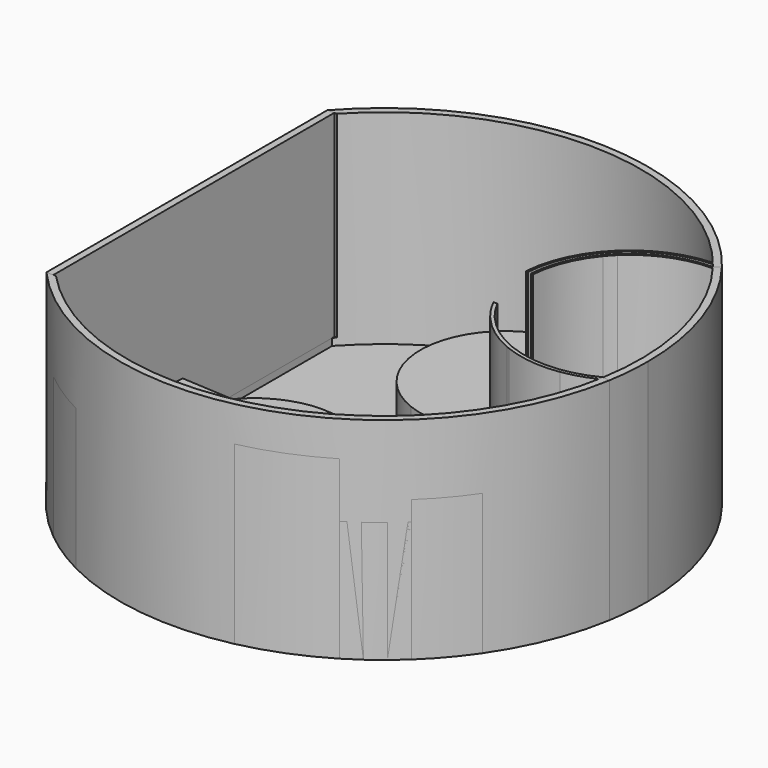
from build123d import *

# Parameters (mm, degrees)
F0_R         = 37.5
F1_DEPTH     = 30
F3_DEPTH     = 28
F8_T         = 1
F8_T3_DEPTH  = 51.8898787331
F9_DEPTH     = 20
F10_DEPTH    = 20
F11_DEPTH    = 25
F12_DEPTH    = 25
F13_DEPTH    = 30
F14_DEPTH    = 30
F15_DEPTH    = 20
F16_DEPTH    = 20
F17_W        = 49.8898787331
F17_H        = 28
F18_DEPTH    = 1.3551748111
F19_DEPTH    = 1
F22_DEPTH    = 5
F23_DEPTH    = 10
F24_DEPTH    = 9
F25_DEPTH    = 8
F26_DEPTH    = 30
F27_DEPTH    = 6
F28_DEPTH    = 4
F21_R        = 1
F29_DEPTH    = 10.5
F30_DEPTH    = 11
F31_DEPTH    = 10
F32_DEPTH    = 8
F33_DEPTH    = 25
F34_DEPTH    = 25
F35_T2_ANGLE = 246.718091376


# Not quite as in the source:
# - a fillet or chamfer that OpenCascade refuses, or shapes differently, is made with other operations: its cross-section is extruded or revolved along the edge and cut away or added
# - a shell that OpenCascade refuses in one call is made with other operations: the cavity is built on its own and cut out


with BuildPart() as f1:
    # F0 (on Top) → F1 (new body)
    with BuildSketch(Plane.XY):
        Circle(F0_R)
    extrude(amount=-F1_DEPTH)

    # F2 (on face) → F3 (cut)
    with BuildSketch(Plane.XY):
        with BuildLine():
            Line((-28, -24.9449393665), (-28, 24.9449393665))
            ThreePointArc((-28, 24.9449393665), (-37.5, 0), (-28, -24.9449393665))
        make_face()
    extrude(amount=-F3_DEPTH, mode=Mode.SUBTRACT)

    # F8: shell of thickness 1, made by hand


with BuildPart() as f8_core1:
    # F8_t2: copy of F1
    add(f1.part)

    # the walls: a layer under each face that stays
    f8_faces = [f8_core1.faces().sort_by_distance(p)[0] for p in [
        (18.75, 32.4759526419, -25),
        (-28, 0, -14),
        (-32.75, 0, -28),
        (0, 0, -30),
    ]]
    thicken(f8_faces, amount=-F8_T, mode=Mode.SUBTRACT)

    # F8_s4 → F8_t3 (cut)
    with BuildSketch(Plane.XZ.offset(-25.9449393665)):
        Polygon((-28.01, -27.99), (-27, -28), (-27, -29), (-28, -29), align=None)
    extrude(amount=F8_T3_DEPTH, mode=Mode.SUBTRACT)


with BuildPart() as f1_1:
    add(f1.part)

    # what is left inside the walls is the cavity
    f8_cavity = [f8_core1.part.solids().sort_by_distance(p)[0] for p in [
        (36.49, 0, -19.333333),
    ]]
    add(f8_cavity, mode=Mode.SUBTRACT)

    # F6 (on face) → F9 (cut)
    with BuildSketch(Plane(origin=(0, 0, -30), x_dir=(1, 0, 0), z_dir=(0, 0, -1))):
        with BuildLine():
            ThreePointArc((-16.953998922, 33.4486460197), (-20.4251291644, 31.4493894793), (-23.6632020109, 29.0912851313))
            Line((-23.6632020109, 29.0912851313), (-23.0321832906, 28.3155175278))
            ThreePointArc((-23.0321832906, 28.3155175278), (-19.8804590533, 30.6107390931), (-16.501892284, 32.5566821259))
            Line((-16.501892284, 32.5566821259), (-16.953998922, 33.4486460197))
        make_face()
    extrude(amount=-F9_DEPTH, mode=Mode.SUBTRACT)

    # F7 (on face) → F11 (cut)
    with BuildSketch(Plane(origin=(0, 0, -30), x_dir=(1, 0, 0), z_dir=(0, 0, -1))):
        with BuildLine():
            ThreePointArc((19.3711654827, 32.1093124785), (13.8934103709, 34.8313529491), (8.046001078, 36.6266551387))
            Line((8.046001078, 36.6266551387), (6.8659209199, 31.2547457184))
            ThreePointArc((6.8659209199, 31.2547457184), (11.2981173091, 29.9391473704), (15.494474725, 27.9985937682))
            Line((15.494474725, 27.9985937682), (19.3711654827, 32.1093124785))
        make_face()
    extrude(amount=-F11_DEPTH, mode=Mode.SUBTRACT)

    # F7 (on face) → F13 (cut)
    with BuildSketch(Plane(origin=(0, 0, -30), x_dir=(1, 0, 0), z_dir=(0, 0, -1))):
        with BuildLine():
            Line((28.9052016216, -22.2876494771), (29.6971249537, -22.8982700107))
            ThreePointArc((29.6971249537, -22.8982700107), (35.49571936, -12.0956152021), (37.5, 0))
            ThreePointArc((37.5, 0), (37.3706102437, 3.1124732958), (36.9833338658, 6.2034680763))
            Line((36.9833338658, 6.2034680763), (35.9971116293, 6.038042261))
            ThreePointArc((35.9971116293, 6.038042261), (35.4071146726, -8.8648875097), (28.9052016216, -22.2876494771))
        make_face()
    extrude(amount=-F13_DEPTH, mode=Mode.SUBTRACT)

    # F7 (on face) → F15 (cut)
    with BuildSketch(Plane(origin=(0, 0, -30), x_dir=(1, 0, 0), z_dir=(0, 0, -1))):
        with BuildLine():
            ThreePointArc((30.9299683404, 21.2034680763), (28.4918045576, 24.3816954507), (25.7285399775, 27.2817197153))
            Line((25.7285399775, 27.2817197153), (25.0424455781, 26.5542071896))
            ThreePointArc((25.0424455781, 26.5542071896), (27.7320231027, 23.7315169054), (30.1051691846, 20.638042261))
            Line((30.1051691846, 20.638042261), (30.9299683404, 21.2034680763))
        make_face()
    extrude(amount=-F15_DEPTH, mode=Mode.SUBTRACT)

    # F17 (on face) → F18 (cut, through all)
    with BuildSketch(Plane(origin=(-28, 0, 0), x_dir=(0, -1, 0), z_dir=(-1, 0, 0))):
        with Locations((0, -14)):
            Rectangle(F17_W, F17_H)
    extrude(amount=-F18_DEPTH, mode=Mode.SUBTRACT)


with BuildPart() as f10:
    # F6 (on face) → F10 (new body)
    with BuildSketch(Plane(origin=(0, 0, -30), x_dir=(1, 0, 0), z_dir=(0, 0, -1))):
        with BuildLine():
            ThreePointArc((-16.953998922, 33.4486460197), (-20.4251291644, 31.4493894793), (-23.6632020109, 29.0912851313))
            Line((-23.6632020109, 29.0912851313), (-23.0321832906, 28.3155175278))
            ThreePointArc((-23.0321832906, 28.3155175278), (-19.8804590533, 30.6107390931), (-16.501892284, 32.5566821259))
            Line((-16.501892284, 32.5566821259), (-16.953998922, 33.4486460197))
        make_face()
    extrude(amount=-F10_DEPTH)


with BuildPart() as f12:
    # F7 (on face) → F12 (new body)
    with BuildSketch(Plane(origin=(0, 0, -30), x_dir=(1, 0, 0), z_dir=(0, 0, -1))):
        with BuildLine():
            ThreePointArc((19.3711654827, 32.1093124785), (13.8934103709, 34.8313529491), (8.046001078, 36.6266551387))
            Line((8.046001078, 36.6266551387), (6.8659209199, 31.2547457184))
            ThreePointArc((6.8659209199, 31.2547457184), (11.2981173091, 29.9391473704), (15.494474725, 27.9985937682))
            Line((15.494474725, 27.9985937682), (19.3711654827, 32.1093124785))
        make_face()
    extrude(amount=-F12_DEPTH)


with BuildPart() as f14:
    # F7 (on face) → F14 (new body)
    with BuildSketch(Plane(origin=(0, 0, -30), x_dir=(1, 0, 0), z_dir=(0, 0, -1))):
        with BuildLine():
            Line((28.9052016216, -22.2876494771), (29.6971249537, -22.8982700107))
            ThreePointArc((29.6971249537, -22.8982700107), (35.49571936, -12.0956152021), (37.5, 0))
            ThreePointArc((37.5, 0), (37.3706102437, 3.1124732958), (36.9833338658, 6.2034680763))
            Line((36.9833338658, 6.2034680763), (35.9971116293, 6.038042261))
            ThreePointArc((35.9971116293, 6.038042261), (35.4071146726, -8.8648875097), (28.9052016216, -22.2876494771))
        make_face()
    extrude(amount=-F14_DEPTH)


with BuildPart() as f16:
    # F7 (on face) → F16 (new body)
    with BuildSketch(Plane(origin=(0, 0, -30), x_dir=(1, 0, 0), z_dir=(0, 0, -1))):
        with BuildLine():
            ThreePointArc((30.9299683404, 21.2034680763), (28.4918045576, 24.3816954507), (25.7285399775, 27.2817197153))
            Line((25.7285399775, 27.2817197153), (25.0424455781, 26.5542071896))
            ThreePointArc((25.0424455781, 26.5542071896), (27.7320231027, 23.7315169054), (30.1051691846, 20.638042261))
            Line((30.1051691846, 20.638042261), (30.9299683404, 21.2034680763))
        make_face()
    extrude(amount=-F16_DEPTH)


with BuildPart() as f19:
    # F17 (on face) → F19 (new body)
    with BuildSketch(Plane(origin=(-28, 0, 0), x_dir=(0, -1, 0), z_dir=(-1, 0, 0))):
        with Locations((0, -14)):
            Rectangle(F17_W, F17_H)
    extrude(amount=-F19_DEPTH)


with BuildPart() as f22:
    # F20 (on face) → F22 (new body)
    with BuildSketch(Plane(origin=(0, 0, -30), x_dir=(1, 0, 0), z_dir=(0, 0, -1))):
        with BuildLine():
            ThreePointArc((-6.2381378075, -12.6227108912), (-8.6582514015, -33.9201866001), (10.2955201074, -23.9104929502))
            ThreePointArc((10.2955201074, -23.9104929502), (9.929155312, -20.9530515767), (8.8522099626, -18.1744059794))
            ThreePointArc((8.8522099626, -18.1744059794), (2.3602210357, -12.5358422681), (-6.2381378075, -12.6227108912))
        make_face()
    extrude(amount=-F22_DEPTH)


with BuildPart() as f22b:
    # F20 (on face) → F22, piece 2 (new body)
    with BuildSketch(Plane(origin=(0, 0, -30), x_dir=(1, 0, 0), z_dir=(0, 0, -1))):
        with BuildLine():
            ThreePointArc((-2.6626795947, 11.4102402329), (-24.8517523428, 10.5323016938), (-9.1514433618, -5.1720296642))
            ThreePointArc((-9.1514433618, -5.1720296642), (-3.5554076268, -0.7180191141), (-1.4451012766, 6.1157523948))
            ThreePointArc((-1.4451012766, 6.1157523948), (-1.7534174258, 8.8320963728), (-2.6626795947, 11.4102402329))
        make_face()
    extrude(amount=-F22_DEPTH)


with BuildPart() as f22c:
    # F20 (on face) → F22, piece 3 (new body)
    with BuildSketch(Plane(origin=(0, 0, -30), x_dir=(1, 0, 0), z_dir=(0, 0, -1))):
        with BuildLine():
            Line((9.0313370609, 9.5891463299), (9.0313370609, 11.6807336927))
            ThreePointArc((9.0313370609, 11.6807336927), (6.9616271493, 12.092424591), (5.2070118097, 13.2648210787))
            Line((5.2070118097, 13.2648210787), (3.728036202, 11.785845471))
            ThreePointArc((3.728036202, 11.785845471), (6.1612113182, 10.1600498361), (9.0313370609, 9.5891463299))
        make_face()
    extrude(amount=-F22_DEPTH)


with BuildPart() as f22d:
    # F20 (on face) → F22, piece 4 (new body)
    with BuildSketch(Plane(origin=(0, 0, -30), x_dir=(1, 0, 0), z_dir=(0, 0, -1))):
        with BuildLine():
            Line((12.8556623122, 13.2648210787), (14.3346379198, 11.785845471))
            ThreePointArc((14.3346379198, 11.785845471), (15.9604335548, 14.2190205872), (16.5313370609, 17.0891463299))
            Line((16.5313370609, 17.0891463299), (14.4397496982, 17.0891463299))
            ThreePointArc((14.4397496982, 17.0891463299), (14.0280587999, 15.0194364182), (12.8556623122, 13.2648210787))
        make_face()
    extrude(amount=-F22_DEPTH)


with BuildPart() as f22e:
    # F20 (on face) → F22, piece 5 (new body)
    with BuildSketch(Plane(origin=(0, 0, -30), x_dir=(1, 0, 0), z_dir=(0, 0, -1))):
        with BuildLine():
            ThreePointArc((9.0313370609, 22.4975589671), (11.1010469726, 22.0858680688), (12.8556623122, 20.9134715811))
            Line((12.8556623122, 20.9134715811), (14.3346379198, 22.3924471888))
            ThreePointArc((14.3346379198, 22.3924471888), (11.9014628037, 24.0182428237), (9.0313370609, 24.5891463299))
            Line((9.0313370609, 24.5891463299), (9.0313370609, 22.4975589671))
        make_face()
    extrude(amount=-F22_DEPTH)


with BuildPart() as f22f:
    # F20 (on face) → F22, piece 6 (new body)
    with BuildSketch(Plane(origin=(0, 0, -30), x_dir=(1, 0, 0), z_dir=(0, 0, -1))):
        with BuildLine():
            ThreePointArc((3.6229244237, 17.0891463299), (4.034615322, 19.1588562416), (5.2070118097, 20.9134715811))
            Line((5.2070118097, 20.9134715811), (3.728036202, 22.3924471888))
            ThreePointArc((3.728036202, 22.3924471888), (2.1022405671, 19.9592720726), (1.5313370609, 17.0891463299))
            Line((1.5313370609, 17.0891463299), (3.6229244237, 17.0891463299))
        make_face()
    extrude(amount=-F22_DEPTH)


with BuildPart() as f23:
    # F20 (on face) → F23 (new body)
    with BuildSketch(Plane(origin=(0, 0, -30), x_dir=(1, 0, 0), z_dir=(0, 0, -1))):
        with BuildLine():
            ThreePointArc((14.0313370609, 17.0891463299), (7.9107331096, 21.9619531991), (4.5336383473, 14.9049516772))
            ThreePointArc((4.5336383473, 14.9049516772), (10.1519410123, 12.2163394607), (14.0313370609, 17.0891463299))
        make_face()
    extrude(amount=-F23_DEPTH)


with BuildPart() as f24:
    # F21 (on face) → F24 (new body)
    with BuildSketch(Plane(origin=(0, 0, -30), x_dir=(1, 0, 0), z_dir=(0, 0, -1))):
        with BuildLine():
            ThreePointArc((-13.6560176054, 7.6129946), (-12.5370872916, 7.2080835014), (-12.0651012766, 6.1157523948))
            ThreePointArc((-12.0651012766, 6.1157523948), (-12.472770206, 5.0877383715), (-13.4741850526, 4.6185101832))
            Line((-13.4741850526, 4.6185101832), (-1.4694765849, 5.3474664352))
            Line((-1.4694765849, 5.3474664352), (-1.6513092498, 8.3419508452))
            Line((-1.6513092498, 8.3419508452), (-13.6560176054, 7.6129946))
        make_face()
    extrude(amount=-F24_DEPTH)


with BuildPart() as f24b:
    # F21 (on face) → F24, piece 2 (new body)
    with BuildSketch(Plane(origin=(0, 0, -30), x_dir=(1, 0, 0), z_dir=(0, 0, -1))):
        with BuildLine():
            ThreePointArc((-13.4741850526, 4.6185101832), (-15.0623434851, 6.0248361184), (-13.6560176054, 7.6129946))
            Line((-13.6560176054, 7.6129946), (-25.6607259684, 6.8840383544))
            Line((-25.6607259684, 6.8840383544), (-25.4788933035, 3.8895539444))
            Line((-25.4788933035, 3.8895539444), (-13.4741850526, 4.6185101832))
        make_face()
    extrude(amount=-F24_DEPTH)


with BuildPart() as f25:
    # F21 (on face) → F25 (new body)
    with BuildSketch(Plane(origin=(0, 0, -30), x_dir=(1, 0, 0), z_dir=(0, 0, -1))):
        with BuildLine():
            ThreePointArc((-13.4741850526, 4.6185101832), (-12.472770206, 5.0877383715), (-12.0651012766, 6.1157523948))
            ThreePointArc((-12.0651012766, 6.1157523948), (-12.5370872916, 7.2080835014), (-13.6560176054, 7.6129946))
            ThreePointArc((-13.6560176054, 7.6129946), (-15.0623434851, 6.0248361184), (-13.4741850526, 4.6185101832))
        make_face()
    extrude(amount=-F25_DEPTH)


with BuildPart() as f26:
    # F21 (on face) → F26 (new body)
    with BuildSketch(Plane(origin=(0, 0, -30), x_dir=(1, 0, 0), z_dir=(0, 0, -1))):
        with BuildLine():
            Line((17.3724938816, 2.8304197599), (17.0417262015, 2.4334684989))
            ThreePointArc((17.0417262015, 2.4334684989), (16.0363047925, 1.0321677906), (15.1927880508, -0.4721577696))
            Line((15.1927880508, -0.4721577696), (15.7749208381, -0.4269615575))
            ThreePointArc((15.7749208381, -0.4269615575), (16.5120762756, 0.8478783333), (17.3706855082, 2.0442917535))
            ThreePointArc((17.3706855082, 2.0442917535), (17.5291229842, 2.2402246522), (17.6908293548, 2.4334684989))
            ThreePointArc((17.6908293548, 2.4334684989), (20.2548787509, 4.8158309177), (23.3012175242, 6.5391475102))
            ThreePointArc((23.3012175242, 6.5391475102), (23.5343220983, 6.634826098), (23.7690009761, 6.7265755334))
            ThreePointArc((23.7690009761, 6.7265755334), (29.9565305021, 7.6871850383), (35.9971116293, 6.038042261))
            Line((35.9971116293, 6.038042261), (35.8888105379, 6.6515620853))
            ThreePointArc((35.8888105379, 6.6515620853), (33.7046086375, 7.5152810001), (31.4149776339, 8.039054017))
            ThreePointArc((31.4149776339, 8.039054017), (27.3986887439, 8.1157854532), (23.4975592214, 7.157843592))
            Line((23.4975592214, 7.157843592), (23.019151936, 6.9626410533))
            ThreePointArc((23.019151936, 6.9626410533), (19.9595995404, 5.2193283623), (17.3724938816, 2.8304197599))
        make_face()
    extrude(amount=-F26_DEPTH)


with BuildPart() as f26b:
    # F21 (on face) → F26, piece 2 (new body)
    with BuildSketch(Plane(origin=(0, 0, -30), x_dir=(1, 0, 0), z_dir=(0, 0, -1))):
        with BuildLine():
            ThreePointArc((18.9043539971, -17.8658754357), (18.9379553483, -18.1056753585), (18.9756990746, -18.3448582694))
            ThreePointArc((18.9756990746, -18.3448582694), (23.5775248273, -21.2302434033), (28.9052016216, -22.2876494771))
            Line((28.9052016216, -22.2876494771), (29.1132550673, -21.9890924211))
            ThreePointArc((29.1132550673, -21.9890924211), (23.6081987695, -20.9193659017), (18.9043539971, -17.8658754357))
        make_face()
        with BuildLine():
            ThreePointArc((14.1582603233, -8.4501833766), (15.2874731924, -13.1069748149), (17.8275811834, -17.1700622615))
            ThreePointArc((17.8275811834, -17.1700622615), (17.8109483721, -16.9218415031), (17.7984344878, -16.673379035))
            ThreePointArc((17.7984344878, -16.673379035), (15.4889985638, -12.8090231025), (14.4573602182, -8.4269615575))
            Line((14.4573602182, -8.4269615575), (14.1582603233, -8.4501833766))
        make_face()
        with BuildLine():
            ThreePointArc((17.7984344878, -16.673379035), (17.8109483721, -16.9218415031), (17.8275811834, -17.1700622615))
            Line((17.8275811834, -17.1700622615), (18.9756990746, -18.3448582694))
            ThreePointArc((18.9756990746, -18.3448582694), (18.9379553483, -18.1056753585), (18.9043539971, -17.8658754357))
            ThreePointArc((18.9043539971, -17.8658754357), (18.3348896843, -17.2849335397), (17.7984344878, -16.673379035))
        make_face()
    extrude(amount=-F26_DEPTH)


with BuildPart() as f26c:
    # F21 (on face) → F26, piece 3 (new body)
    with BuildSketch(Plane(origin=(0, 0, -30), x_dir=(1, 0, 0), z_dir=(0, 0, -1))):
        with BuildLine():
            Line((28.2867848352, -23.0674620122), (28.5205850004, -22.7777573794))
            ThreePointArc((28.5205850004, -22.7777573794), (18.3702197288, -18.4621489283), (13.6597604985, -8.4888864085))
            Line((13.6597604985, -8.4888864085), (13.3606606036, -8.5121082276))
            ThreePointArc((13.3606606036, -8.5121082276), (18.0823472399, -18.6009920186), (28.2867848352, -23.0674620122))
        make_face()
    extrude(amount=-F26_DEPTH)


with BuildPart() as f27:
    # F21 (on face) → F27 (new body)
    with BuildSketch(Plane(origin=(0, 0, -30), x_dir=(1, 0, 0), z_dir=(0, 0, -1))):
        with BuildLine():
            ThreePointArc((36.4690616321, -1.5025124541), (23.3259292755, -4.4017029134), (17.7984344878, -16.673379035))
            ThreePointArc((17.7984344878, -16.673379035), (18.3348896843, -17.2849335397), (18.9043539971, -17.8658754357))
            ThreePointArc((18.9043539971, -17.8658754357), (23.5577123643, -5.5144047174), (36.4128165524, -2.521267682))
            Line((36.4128165524, -2.521267682), (36.4690616321, -1.5025124541))
        make_face()
    extrude(amount=-F27_DEPTH)


with BuildPart() as f28:
    # F21 (on face) → F28 (new body)
    with BuildSketch(Plane(origin=(0, 0, -30), x_dir=(1, 0, 0), z_dir=(0, 0, -1))):
        with BuildLine():
            Line((33.6939781628, 0.0919253308), (33.384353908, 4.0799239292))
            Line((33.384353908, 4.0799239292), (30.3933549592, 3.8477057381))
            ThreePointArc((30.3933549592, 3.8477057381), (28.5541677874, 1.6988943115), (30.7029792141, -0.1402928603))
            Line((30.7029792141, -0.1402928603), (33.6939781628, 0.0919253308))
        make_face()
    extrude(amount=-F28_DEPTH)


with BuildPart() as f29:
    # F21 (on face) → F29 (new body)
    with BuildSketch(Plane(origin=(0, 0, -30), x_dir=(1, 0, 0), z_dir=(0, 0, -1))):
        with Locations((28.4533989432, 12.6025223553)):
            Circle(F21_R)
    extrude(amount=-F29_DEPTH)


with BuildPart() as f29b:
    # F21 (on face) → F29, piece 2 (new body)
    with BuildSketch(Plane(origin=(0, 0, -30), x_dir=(1, 0, 0), z_dir=(0, 0, -1))):
        with Locations((29.3880372101, 17.2326898803)):
            Circle(F21_R)
    extrude(amount=-F29_DEPTH)


with BuildPart() as f29c:
    # F21 (on face) → F29, piece 3 (new body)
    with BuildSketch(Plane(origin=(0, 0, -30), x_dir=(1, 0, 0), z_dir=(0, 0, -1))):
        with Locations((26.1902851373, 14.5718663836)):
            Circle(F21_R)
    extrude(amount=-F29_DEPTH)


with BuildPart() as f29d:
    # F21 (on face) → F29, piece 4 (new body)
    with BuildSketch(Plane(origin=(0, 0, -30), x_dir=(1, 0, 0), z_dir=(0, 0, -1))):
        with Locations((30.9132082299, 14.6493096605)):
            Circle(F21_R)
    extrude(amount=-F29_DEPTH)


with BuildPart() as f30:
    # F21 (on face) → F30 (new body)
    with BuildSketch(Plane(origin=(0, 0, -30), x_dir=(1, 0, 0), z_dir=(0, 0, -1))):
        Polygon((35.707328978, -0.0025124541), (35.3590016913, 4.4839859691), (33.3650023921, 4.3291738416), (33.384353908, 4.0799239292), (33.6939781628, 0.0919253308), (33.7133296788, -0.1573245816), align=None)
    extrude(amount=-F30_DEPTH)


with BuildPart() as f31:
    # F21 (on face) → F31 (new body)
    with BuildSketch(Plane(origin=(0, 0, -30), x_dir=(1, 0, 0), z_dir=(0, 0, -1))):
        with BuildLine():
            ThreePointArc((23.4975592214, 7.157843592), (22.5012598633, 8.1254792219), (21.2341408526, 8.6941096256))
            ThreePointArc((21.2341408526, 8.6941096256), (16.9312552069, 7.0414828531), (17.0417262015, 2.4334684989))
            ThreePointArc((17.0417262015, 2.4334684989), (17.2054558605, 2.6333225093), (17.3724938816, 2.8304197599))
            ThreePointArc((17.3724938816, 2.8304197599), (18.1879242771, 7.6403130301), (23.019151936, 6.9626410533))
            ThreePointArc((23.019151936, 6.9626410533), (23.2575421278, 7.0622359485), (23.4975592214, 7.157843592))
        make_face()
        with BuildLine():
            ThreePointArc((34.8341776522, 10.9009204792), (32.9971119, 15.6025833201), (30.5289475825, 20.005833137))
            ThreePointArc((30.5289475825, 20.005833137), (24.4077425239, 15.5609894801), (21.2341408526, 8.6941096256))
            ThreePointArc((21.2341408526, 8.6941096256), (22.5012598633, 8.1254792219), (23.4975592214, 7.157843592))
            ThreePointArc((23.4975592214, 7.157843592), (27.3986887439, 8.1157854532), (31.4149776339, 8.039054017))
            ThreePointArc((31.4149776339, 8.039054017), (32.7879027838, 9.8722277789), (34.8341776522, 10.9009204792))
        make_face()
        with Locations((26.1902851373, 14.5718663836)):
            Circle(F21_R, mode=Mode.SUBTRACT)
        with Locations((28.4533989432, 12.6025223553)):
            Circle(F21_R, mode=Mode.SUBTRACT)
        with Locations((30.9132082299, 14.6493096605)):
            Circle(F21_R, mode=Mode.SUBTRACT)
        with Locations((29.3880372101, 17.2326898803)):
            Circle(F21_R, mode=Mode.SUBTRACT)
    extrude(amount=-F31_DEPTH)


with BuildPart() as f31b:
    # F21 (on face) → F31, piece 2 (new body)
    with BuildSketch(Plane(origin=(0, 0, -30), x_dir=(1, 0, 0), z_dir=(0, 0, -1))):
        with BuildLine():
            ThreePointArc((17.3706855082, 2.0442917535), (22.6171124353, 1.5878513607), (23.7690009761, 6.7265755334))
            Line((23.7690009761, 6.7265755334), (23.3012175242, 6.5391475102))
            ThreePointArc((23.3012175242, 6.5391475102), (22.3218332247, 1.9913488053), (17.6908293548, 2.4334684989))
            Line((17.6908293548, 2.4334684989), (17.3706855082, 2.0442917535))
        make_face()
    extrude(amount=-F31_DEPTH)


with BuildPart() as f32:
    # F21 (on face) → F32 (new body)
    with BuildSketch(Plane(origin=(0, 0, -30), x_dir=(1, 0, 0), z_dir=(0, 0, -1))):
        with BuildLine():
            ThreePointArc((23.019151936, 6.9626410533), (18.1879242771, 7.6403130301), (17.3724938816, 2.8304197599))
            ThreePointArc((17.3724938816, 2.8304197599), (19.9595995404, 5.2193283623), (23.019151936, 6.9626410533))
        make_face()
    extrude(amount=-F32_DEPTH)


with BuildPart() as f32b:
    # F21 (on face) → F32, piece 2 (new body)
    with BuildSketch(Plane(origin=(0, 0, -30), x_dir=(1, 0, 0), z_dir=(0, 0, -1))):
        with BuildLine():
            ThreePointArc((17.6908293548, 2.4334684989), (22.3218332247, 1.9913488053), (23.3012175242, 6.5391475102))
            ThreePointArc((23.3012175242, 6.5391475102), (20.2548787509, 4.8158309177), (17.6908293548, 2.4334684989))
        make_face()
    extrude(amount=-F32_DEPTH)


with BuildPart() as f33:
    # F21 (on face) → F33 (new body)
    with BuildSketch(Plane(origin=(0, 0, -30), x_dir=(1, 0, 0), z_dir=(0, 0, -1))):
        with BuildLine():
            ThreePointArc((35.8888105379, 6.6515620853), (35.4252667785, 8.7920687938), (34.8341776522, 10.9009204792))
            ThreePointArc((34.8341776522, 10.9009204792), (32.7879027838, 9.8722277789), (31.4149776339, 8.039054017))
            ThreePointArc((31.4149776339, 8.039054017), (33.7046086375, 7.5152810001), (35.8888105379, 6.6515620853))
        make_face()
    extrude(amount=-F33_DEPTH)


with BuildPart() as f34:
    # F7 (on face) → F34 (new body)
    with BuildSketch(Plane(origin=(0, 0, -30), x_dir=(1, 0, 0), z_dir=(0, 0, -1))):
        with BuildLine():
            ThreePointArc((25.7285399775, 27.2817197153), (22.6786743687, 29.8651591135), (19.3711654827, 32.1093124785))
            Line((19.3711654827, 32.1093124785), (15.494474725, 27.9985937682))
            ThreePointArc((15.494474725, 27.9985937682), (18.8727717778, 25.8421842232), (21.9550207808, 23.2804008237))
            Line((21.9550207808, 23.2804008237), (25.0424455781, 26.5542071896))
            Line((25.0424455781, 26.5542071896), (25.7285399775, 27.2817197153))
        make_face()
    extrude(amount=-F34_DEPTH)

    # F35: chamfer of 8 x 25 on 1 edges, made by hand

    # F35_s1 → F35_t2 (revolve, cut)
    with BuildSketch(Plane(origin=(0, 0, 0), x_dir=(0, 0, 1), z_dir=(-0.048534848, 0.9988214898, 0))):
        Polygon((-5, -40), (-30, -32), (-5, -32), align=None)
    revolve(axis=Axis((0, 0, -5), (0, 0, 1)), revolution_arc=F35_T2_ANGLE, mode=Mode.SUBTRACT)


solid = Compound([f1_1.part, f10.part, f12.part, f14.part, f16.part, f19.part, f22.part, f22b.part, f22c.part, f22d.part, f22e.part, f22f.part, f23.part, f24.part, f24b.part, f25.part, f26.part, f26b.part, f26c.part, f27.part, f28.part, f29.part, f29b.part, f29c.part, f29d.part, f30.part, f31.part, f31b.part, f32.part, f32b.part, f33.part, f34.part])
